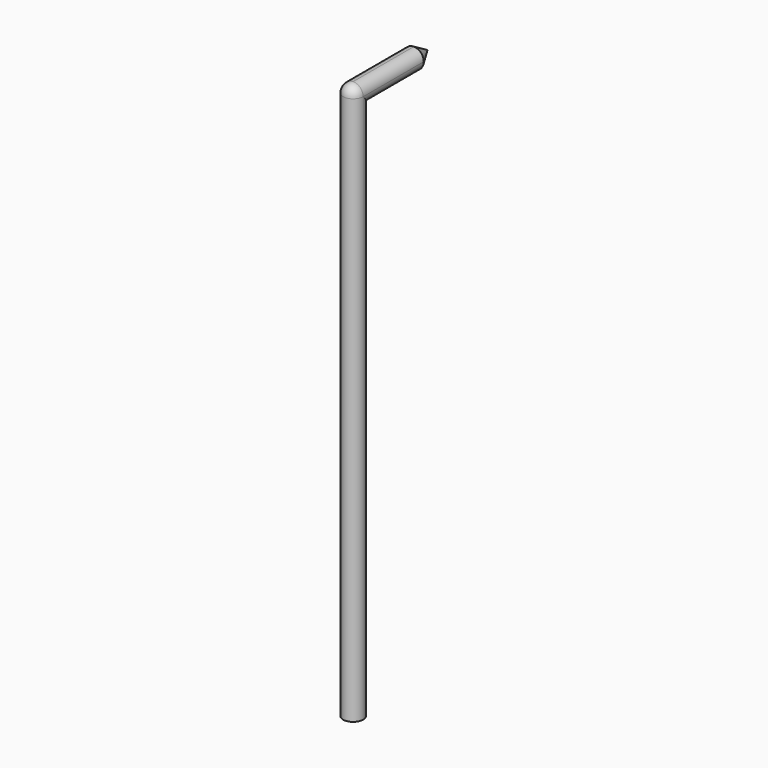
from build123d import *

# Parameters (mm, degrees)
F1_DEPTH     = 42
F2_START     = 40.5
F2_DEPTH     = 1.5
F3_T1_DEPTH  = 8.875
F3_T4_ANGLE  = 180
F3_T8_DEPTH  = 10.75
F3_S9_R      = 0.75
F3_T10_DEPTH = 7
F3_T14_DEPTH = 10.75
F3_S15_R     = 0.75
F3_T16_DEPTH = 7
F4_SIZE2     = 1.299028
F4_SIZE      = 0.74999


# Not quite as in the source:
# - a fillet or chamfer that OpenCascade refuses, or shapes differently, is made with other operations: its cross-section is extruded or revolved along the edge and cut away or added
# - a fillet or chamfer is up to 0.001 mm smaller than in the source, because OpenCascade refuses the exact size


with BuildPart() as f1:
    # F0 (on Top) → F1 (new body)
    with BuildSketch(Plane.XY):
        with BuildLine():
            Line((-0.75, 0), (0.75, 0))
            ThreePointArc((0.75, 0), (0, 0.75), (-0.75, 0))
        make_face()
        with BuildLine():
            ThreePointArc((-0.75, 0), (0, -0.75), (0.75, 0))
            Line((0.75, 0), (-0.75, 0))
        make_face()
    extrude(amount=F1_DEPTH)

    # F0 (on Top) → F2 (join)
    with BuildSketch(Plane.XY.offset(F2_START)):
        with BuildLine():
            ThreePointArc((-0.75, 0), (0, 0.75), (0.75, 0))
            Line((0.75, 0), (0.75, 7))
            Line((0.75, 7), (-0.75, 7))
            Line((-0.75, 7), (-0.75, 0))
        make_face()
    extrude(amount=F2_DEPTH)

    # F3: fillet of radius 0.75 on 5 edges, made by hand

    # F3_s2 → F3_t1 (cut)
    with BuildSketch(Plane.XZ.offset(-8.875)):
        with BuildLine():
            ThreePointArc((0.75, 41.25), (0.5303300859, 41.7803300859), (0, 42))
            Line((0, 42), (0.75, 42))
            Line((0.75, 42), (0.75, 41.25))
        make_face()
        with BuildLine():
            ThreePointArc((0, 42), (-0.5303300859, 41.7803300859), (-0.75, 41.25))
            Line((-0.75, 41.25), (-0.75, 42))
            Line((-0.75, 42), (0, 42))
        make_face()
    extrude(amount=F3_T1_DEPTH, mode=Mode.SUBTRACT)

    # F3_s3 → F3_t4 (revolve, cut)
    with BuildSketch(Plane.XZ):
        with BuildLine():
            ThreePointArc((-0.75, 41.25), (-0.5303300859, 41.7803300859), (0, 42))
            Line((0, 42), (-0.75, 42))
            Line((-0.75, 42), (-0.75, 41.25))
        make_face()
    revolve(axis=Axis((0, 0, 42), (0, 0, 1)), revolution_arc=F3_T4_ANGLE, mode=Mode.SUBTRACT)


with BuildPart() as f3_tool6:
    # F3_s7 → F3_t8 (new body)
    with BuildSketch(Plane.XZ.offset(-8.875)):
        with BuildLine():
            ThreePointArc((0, 40.5), (-0.5303300859, 40.7196699141), (-0.75, 41.25))
            Line((-0.75, 41.25), (-0.75, 40.5))
            Line((-0.75, 40.5), (0, 40.5))
        make_face()
    extrude(amount=F3_T8_DEPTH)

    # F3_s9 → F3_t10 (cut, symmetric)
    with BuildSketch(Plane.XY.offset(40.9)):
        Circle(F3_S9_R)
    extrude(amount=F3_T10_DEPTH, both=True, mode=Mode.SUBTRACT)


with BuildPart() as f1_1:
    add(f1.part)

    # F3_t5: cut F3_tool6
    add(f3_tool6.part, mode=Mode.SUBTRACT)


with BuildPart() as f3_tool12:
    # F3_s13 → F3_t14 (new body)
    with BuildSketch(Plane.XZ.offset(1.875)):
        with BuildLine():
            ThreePointArc((0, 40.5), (0.5303300859, 40.7196699141), (0.75, 41.25))
            Line((0.75, 41.25), (0.75, 40.5))
            Line((0.75, 40.5), (0, 40.5))
        make_face()
    extrude(amount=-F3_T14_DEPTH)

    # F3_s15 → F3_t16 (cut, symmetric)
    with BuildSketch(Plane.XY.offset(40.9)):
        Circle(F3_S15_R)
    extrude(amount=F3_T16_DEPTH, both=True, mode=Mode.SUBTRACT)


with BuildPart() as f1_2:
    add(f1_1.part)

    # F3_t11: cut F3_tool12
    add(f3_tool12.part, mode=Mode.SUBTRACT)

    # F4 (size 0.75 and 1.2990381057 in the source; OpenCascade refuses exactly that, so slightly less here)
    f4_edges = [f1_2.edges().sort_by_distance(p)[0] for p in [
        (-0.53033, 7, 40.71967),
        (0.53033, 7, 40.71967),
        (-0.53033, 7, 41.78033),
        (0.53033, 7, 41.78033),
    ]]
    f4_side = f1_2.faces().sort_by_distance((0, 7, 41.25))[0]
    chamfer(f4_edges, length=F4_SIZE, length2=F4_SIZE2, reference=f4_side)


solid = f1_2.part
